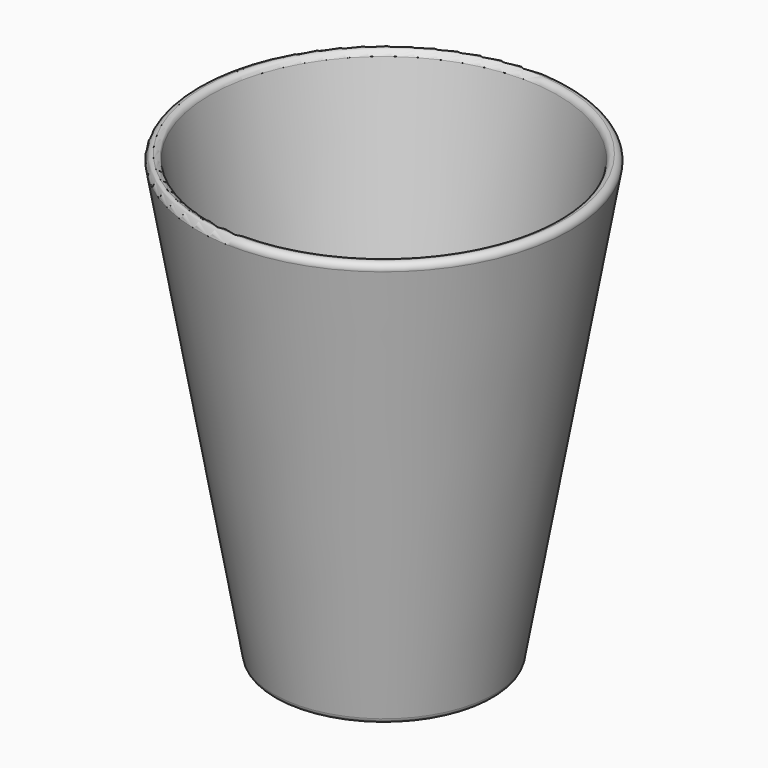
from build123d import *

# Parameters (mm, degrees)
F2_T = -5.08
F3_R = 2.53999
F4_R = 2.54
F5_R = 15.24


# Not quite as in the source:
# - a fillet or chamfer is up to 0.001 mm smaller than in the source, because OpenCascade refuses the exact size


with BuildPart() as f1:
    # F0 (on Front) → F1 (revolve)
    with BuildSketch(Plane.XZ):
        Polygon((-31.75, 3.175), (0, 3.175), (0, 180.975), (-76.2, 180.975), (-44.45, 0), (-38.1, 0), align=None)
    revolve(axis=Axis((0, 0, 92.075), (0, 0, -1)))

    # F2
    f2_openings = [f1.faces().sort_by_distance(p)[0] for p in [
        (0, 0, 180.975),
    ]]
    offset(amount=F2_T, openings=f2_openings, kind=Kind.INTERSECTION)

    # F3 (radius 2.54 in the source; OpenCascade refuses exactly that, so slightly less here)
    f3_edges = [f1.edges().sort_by_distance(p)[0] for p in [
        (76.2, 0, 180.975),
        (71.042415, 0, 180.975),
    ]]
    fillet(f3_edges, radius=F3_R)

    # F4
    f4_edges = [f1.edges().sort_by_distance(p)[0] for p in [
        (44.45, 0, 0),
        (38.1, 0, 0),
    ]]
    fillet(f4_edges, radius=F4_R)

    # F5
    f5_edges = [f1.edges().sort_by_distance(p)[0] for p in [
        (31.75, 0, 3.175),
    ]]
    fillet(f5_edges, radius=F5_R)


solid = f1.part
